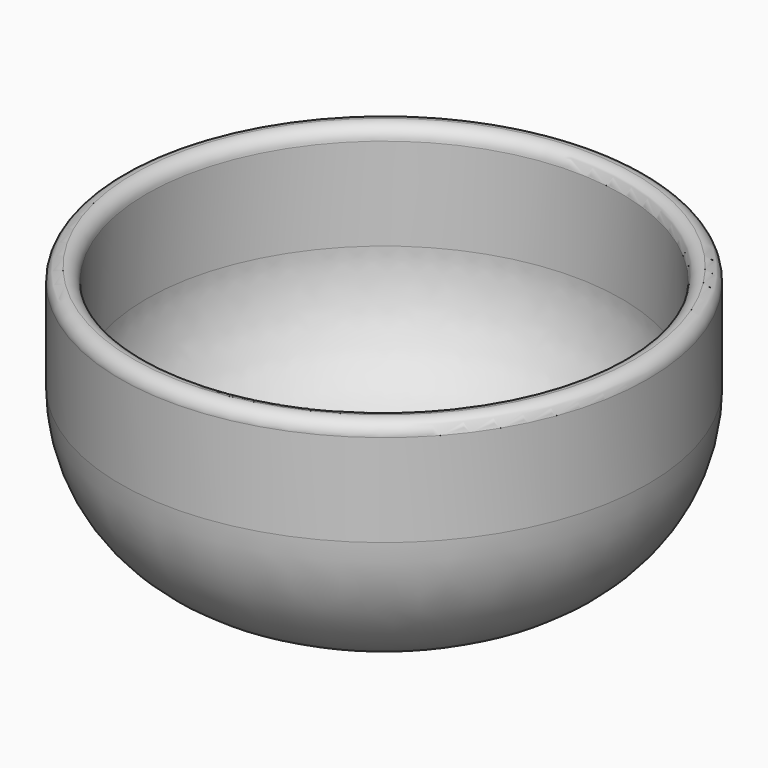
from build123d import *

# Parameters (mm, degrees)
F0_R     = 50
F1_DEPTH = 50
F2_R     = 30
F3_T     = -5
F4_R     = 2.49999


# Not quite as in the source:
# - a fillet or chamfer is up to 0.001 mm smaller than in the source, because OpenCascade refuses the exact size


with BuildPart() as f1:
    # F0 (on Top) → F1 (new body)
    with BuildSketch(Plane.XY):
        Circle(F0_R)
    extrude(amount=F1_DEPTH)

    # F2
    f2_edges = [f1.edges().sort_by_distance(p)[0] for p in [
        (-50, 0, 0),
    ]]
    fillet(f2_edges, radius=F2_R)

    # F3
    f3_openings = [f1.faces().sort_by_distance(p)[0] for p in [
        (0, 0, 50),
    ]]
    offset(amount=F3_T, openings=f3_openings)

    # F4 (radius 2.5 in the source; OpenCascade refuses exactly that, so slightly less here)
    f4_edges = [f1.edges().sort_by_distance(p)[0] for p in [
        (-45, 0, 50),
        (-50, 0, 50),
    ]]
    fillet(f4_edges, radius=F4_R)


solid = f1.part
